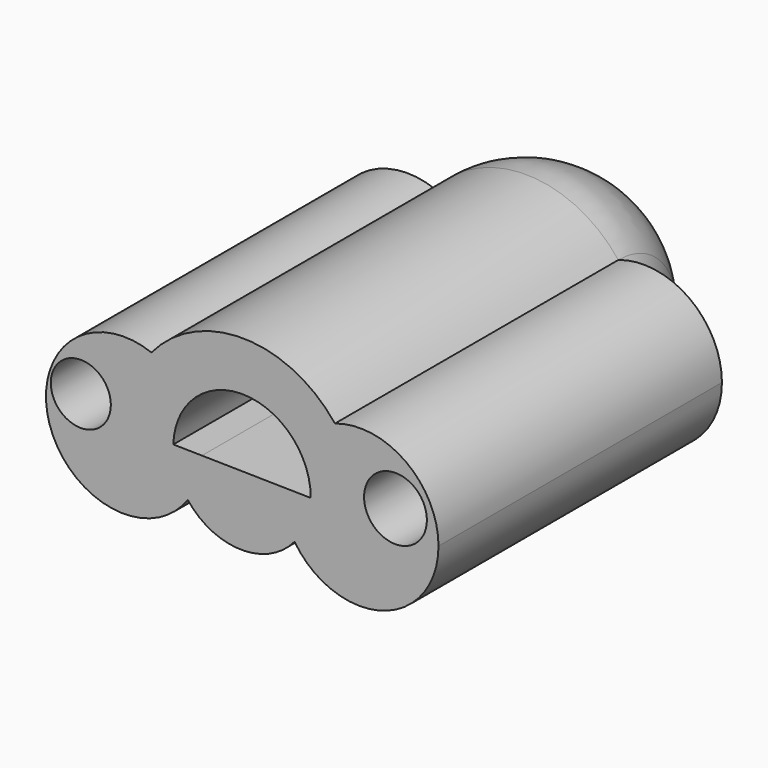
from build123d import *

# Parameters (mm, degrees)
F2_DEPTH = 76.2
F3_R     = 6.7594001511
F3_R_2   = 6.4582232876
F4_DEPTH = 76.2010001


# Not quite as in the source:
# - after a boolean that leaves OpenCascade's solid faulty, fix() repairs it


with BuildPart() as f1:
    # F0 (on Front) → F1 (revolve)
    with BuildSketch(Plane.XZ):
        with BuildLine():
            Line((25.1545395287, 21.3476155531), (35.7739973958, 21.163463243))
            ThreePointArc((35.7739973958, 21.163463243), (34.4297968698, 29.6094722117), (30.3585694498, 37.130579168))
            ThreePointArc((30.3585694498, 37.130579168), (25.6039790041, 34.6113767137), (21.8851704543, 30.722549862))
            ThreePointArc((21.8851704543, 30.722549862), (24.3135197286, 26.3667282707), (25.1549027334, 21.4512286447))
            ThreePointArc((25.1549027334, 21.4512286447), (25.154811932, 21.3994217806), (25.1545395287, 21.3476155531))
        make_face()
        with BuildLine():
            ThreePointArc((21.8851704543, 30.722549862), (25.6039790041, 34.6113767137), (30.3585694498, 37.130579168))
            ThreePointArc((30.3585694498, 37.130579168), (10.7712173211, 46.8481479211), (-9.1092864198, 37.7453419309))
            ThreePointArc((-9.1092864198, 37.7453419309), (-4.4421909583, 35.0671010008), (-0.8631205726, 31.049015673))
            ThreePointArc((-0.8631205726, 31.049015673), (10.5877063894, 36.228982116), (21.8851704543, 30.722549862))
        make_face()
        with BuildLine():
            ThreePointArc((-0.8631205726, 31.049015673), (-4.4421909583, 35.0671010008), (-9.1092864198, 37.7453419309))
            ThreePointArc((-9.1092864198, 37.7453419309), (-13.3970388276, 30.3966371616), (-15.0174490426, 22.0442391088))
            Line((-15.0174490426, 22.0442391088), (-4.3979911756, 21.8600867986))
            ThreePointArc((-4.3979911756, 21.8600867986), (-3.4182084188, 26.7575517121), (-0.8631205726, 31.049015673))
        make_face()
    revolve(axis=Axis((10.3782741766, 0, 21.6038511759), (0.9998496783, 0, -0.0173384207)))

    # F0 (on Front) → F2 (join)
    with BuildSketch(Plane.XZ):
        with BuildLine():
            Line((25.1545395287, 21.3476155531), (35.7739973958, 21.163463243))
            ThreePointArc((35.7739973958, 21.163463243), (34.4297968698, 29.6094722117), (30.3585694498, 37.130579168))
            ThreePointArc((30.3585694498, 37.130579168), (25.6039790041, 34.6113767137), (21.8851704543, 30.722549862))
            ThreePointArc((21.8851704543, 30.722549862), (24.3135197286, 26.3667282707), (25.1549027334, 21.4512286447))
            ThreePointArc((25.1549027334, 21.4512286447), (25.154811932, 21.3994217806), (25.1545395287, 21.3476155531))
        make_face()
        with BuildLine():
            ThreePointArc((30.3585694498, 37.130579168), (34.4297968698, 29.6094722117), (35.7739973958, 21.163463243))
            Line((35.7739973958, 21.163463243), (25.1545395287, 21.3476155531))
            ThreePointArc((25.1545395287, 21.3476155531), (24.2390674494, 16.3295092934), (21.6721533213, 11.9215129889))
            ThreePointArc((21.6721533213, 11.9215129889), (40.5964369904, 5.0073582929), (52.6344733915, 21.163463243))
            ThreePointArc((52.6344733915, 21.163463243), (45.5966487159, 34.8671551487), (30.3585694498, 37.130579168))
        make_face()
        with BuildLine():
            ThreePointArc((21.8851704543, 30.722549862), (25.6039790041, 34.6113767137), (30.3585694498, 37.130579168))
            ThreePointArc((30.3585694498, 37.130579168), (10.7712173211, 46.8481479211), (-9.1092864198, 37.7453419309))
            ThreePointArc((-9.1092864198, 37.7453419309), (-4.4421909583, 35.0671010008), (-0.8631205726, 31.049015673))
            ThreePointArc((-0.8631205726, 31.049015673), (10.5877063894, 36.228982116), (21.8851704543, 30.722549862))
        make_face()
        with BuildLine():
            ThreePointArc((21.6721533213, 11.9215129889), (24.2390674494, 16.3295092934), (25.1545395287, 21.3476155531))
            Line((25.1545395287, 21.3476155531), (18.9160558958, 21.4557972689))
            ThreePointArc((18.9160558958, 21.4557972689), (19.5766912961, 16.4812708171), (21.6721533213, 11.9215129889))
        make_face()
        with BuildLine():
            ThreePointArc((-0.8631205726, 31.049015673), (-4.4421909583, 35.0671010008), (-9.1092864198, 37.7453419309))
            ThreePointArc((-9.1092864198, 37.7453419309), (-13.3970388276, 30.3966371616), (-15.0174490426, 22.0442391088))
            Line((-15.0174490426, 22.0442391088), (-4.3979911756, 21.8600867986))
            ThreePointArc((-4.3979911756, 21.8600867986), (-3.4182084188, 26.7575517121), (-0.8631205726, 31.049015673))
        make_face()
        with BuildLine():
            ThreePointArc((-15.0174490426, 22.0442391088), (-13.3970388276, 30.3966371616), (-9.1092864198, 37.7453419309))
            ThreePointArc((-9.1092864198, 37.7453419309), (-31.0500334974, 17.1058941318), (-1.2989030127, 12.3885407791))
            ThreePointArc((-1.2989030127, 12.3885407791), (-3.6708558605, 16.8552217877), (-4.3979911756, 21.8600867986))
            Line((-4.3979911756, 21.8600867986), (-15.0174490426, 22.0442391088))
        make_face()
        with BuildLine():
            ThreePointArc((21.6721533213, 11.9215129889), (19.5766912961, 16.4812708171), (18.9160558958, 21.4557972689))
            Line((18.9160558958, 21.4557972689), (1.7559349744, 21.7533713965))
            ThreePointArc((1.7559349744, 21.7533713965), (0.9313585185, 16.8416865825), (-1.2989030127, 12.3885407791))
            ThreePointArc((-1.2989030127, 12.3885407791), (10.0752100973, 6.6750070556), (21.6721533213, 11.9215129889))
        make_face()
        with BuildLine():
            ThreePointArc((-4.3979911756, 21.8600867986), (-3.6708558605, 16.8552217877), (-1.2989030127, 12.3885407791))
            ThreePointArc((-1.2989030127, 12.3885407791), (0.9313585185, 16.8416865825), (1.7559349744, 21.7533713965))
            Line((1.7559349744, 21.7533713965), (-4.3979911756, 21.8600867986))
        make_face()
    extrude(amount=F2_DEPTH)

    add(f1.part.fix(), mode=Mode.REPLACE)

    # F3 (on Front) → F4 (cut, through all)
    with BuildSketch(Plane.XZ):
        with Locations((43.3778166771, 25.266315788)):
            Circle(F3_R)
        with Locations((-24.2998190224, 24.9655265361)):
            Circle(F3_R_2)
    extrude(amount=F4_DEPTH, mode=Mode.SUBTRACT)


solid = f1.part
